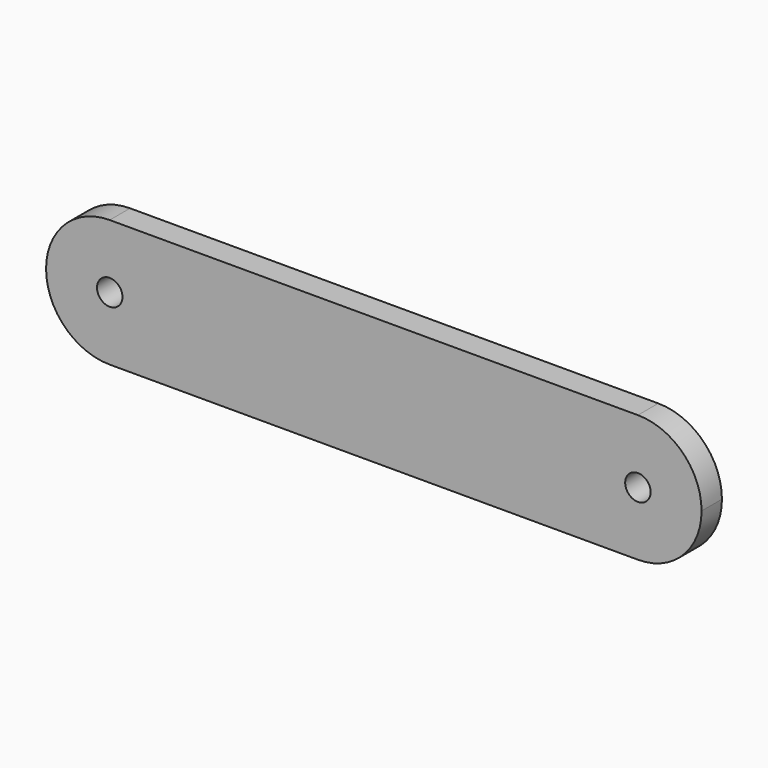
from build123d import *

# Parameters (mm, degrees)
F0_W     = 51.5
F0_H     = 10
F0_R     = 1
F1_DEPTH = 2
F2_R     = 4.99999


# Not quite as in the source:
# - a fillet or chamfer is up to 0.001 mm smaller than in the source, because OpenCascade refuses the exact size


with BuildPart() as f1:
    # F0 (on Front) → F1 (new body)
    with BuildSketch(Plane.XZ):
        with Locations((25.75, -5)):
            Rectangle(F0_W, F0_H)
        with Locations((5, -5)):
            Circle(F0_R, mode=Mode.SUBTRACT)
        with Locations((46.5, -5)):
            Circle(F0_R, mode=Mode.SUBTRACT)
    extrude(amount=F1_DEPTH)

    # F2 (radius 5 in the source; OpenCascade refuses exactly that, so slightly less here)
    f2_edges = [f1.edges().sort_by_distance(p)[0] for p in [
        (0, -1, 0),
        (0, -1, -10),
        (51.5, -1, 0),
        (51.5, -1, -10),
    ]]
    fillet(f2_edges, radius=F2_R)


solid = f1.part
